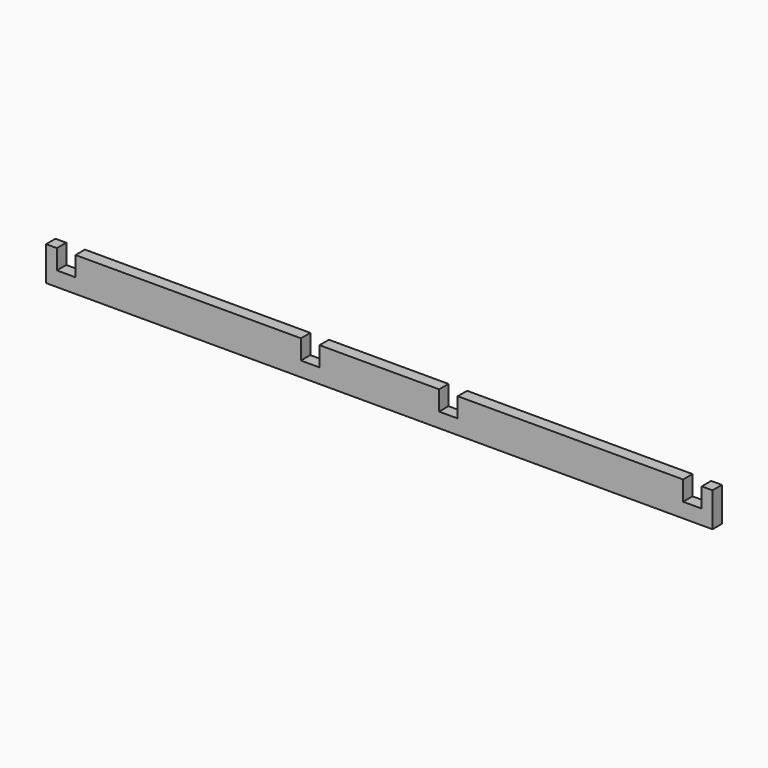
from build123d import *

# Parameters (mm, degrees)
F1_DEPTH = 12


# Not quite as in the source:
# - a feature names something its author has since deleted; it is built from what else it names


with BuildPart() as f1:
    # F0 (on Front) → F1 (new body)
    with BuildSketch(Plane.XZ):
        Polygon((0, 35), (0, 0), (680, 0), (680, 35), (669, 35), (669, 15), (650, 15), (650, 35), (420, 35), (420, 15), (401, 15), (401, 35), (279, 35), (279, 15), (260, 15), (260, 35), (30, 35), (30, 15), (11, 15), (11, 35), align=None)
    extrude(amount=F1_DEPTH)


solid = f1.part
